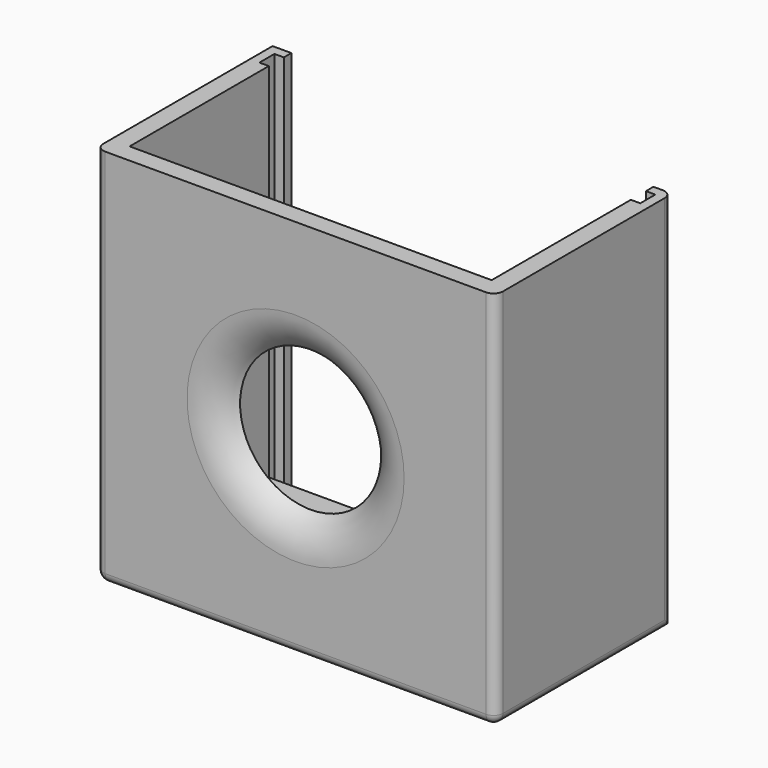
from build123d import *

# Parameters (mm, degrees)
F2_W      = 42.5
F2_H      = 40.5
F2_R      = 7.5
F8_DEPTH  = 2
F6_W      = 23.5
F6_H      = 40.5
F9_DEPTH  = 2
F5_W      = 23.5
F5_H      = 40.5
F10_DEPTH = 2
F0_W      = 42.5
F0_H      = 20.5
F11_DEPTH = 2
F7_W      = 1
F7_H      = 2
F12_DEPTH = 38.5
F13_DEPTH = 40.5
F14_R     = 0.99999


# Not quite as in the source:
# - a fillet or chamfer that OpenCascade refuses, or shapes differently, is made with other operations: its cross-section is extruded or revolved along the edge and cut away or added
# - a fillet or chamfer is up to 0.001 mm smaller than in the source, because OpenCascade refuses the exact size


with BuildPart() as f8:
    # F2 (on line) → F8 (new body)
    with BuildSketch(Plane.XZ.offset(10.25)):
        with Locations((0, 20.25)):
            Rectangle(F2_W, F2_H)
        with Locations((0, 20.25)):
            Circle(F2_R, mode=Mode.SUBTRACT)
    extrude(amount=-F8_DEPTH)

    # F6 (on line) → F9 (join)
    with BuildSketch(Plane(origin=(-21.25, 0, 0), x_dir=(0, -1, 0), z_dir=(-1, 0, 0))):
        with Locations((-1.5, 20.25)):
            Rectangle(F6_W, F6_H)
    extrude(amount=-F9_DEPTH)

    # F5 (on line) → F10 (join)
    with BuildSketch(Plane.YZ.offset(21.25)):
        with Locations((1.5, 20.25)):
            Rectangle(F5_W, F5_H)
    extrude(amount=-F10_DEPTH)

    # F0 (on Top) → F11 (join)
    with BuildSketch(Plane.XY):
        Rectangle(F0_W, F0_H)
    extrude(amount=F11_DEPTH)

    # F7 (on Top) → F12 (cut)
    with BuildSketch(Plane.XY):
        with Locations((-19.75, 11.25)):
            Rectangle(F7_W, F7_H)
        with Locations((19.75, 11.25)):
            Rectangle(F7_W, F7_H)
    extrude(amount=-F12_DEPTH, mode=Mode.SUBTRACT)

    # F7 (on Top) → F13 (cut)
    with BuildSketch(Plane.XY):
        with Locations((19.75, 11.25)):
            Rectangle(F7_W, F7_H)
        with Locations((-19.75, 11.25)):
            Rectangle(F7_W, F7_H)
    extrude(amount=F13_DEPTH, mode=Mode.SUBTRACT)

    # F14 (radius 1 in the source; OpenCascade refuses exactly that, so slightly less here)
    f14_edges = [f8.edges().sort_by_distance(p)[0] for p in [
        (0, -10.25, 0),
        (21.25, 1.5, 0),
        (21.25, 13.25, 20.25),
        (21.25, -10.25, 20.25),
        (-21.25, -10.25, 20.25),
        (-21.25, 1.5, 0),
    ]]
    fillet(f14_edges, radius=F14_R)

    # F15: fillet of radius 5.08 on 1 edges, made by hand

    # F15_s1 → F15_t2 (revolve, cut)
    with BuildSketch(Plane.XY.offset(20.25)):
        with BuildLine():
            ThreePointArc((11.5398019753, -10.25), (9.2859164414, -9.7226256161), (7.5, -8.25))
            Line((7.5, -8.25), (7.5, -10.25))
            Line((7.5, -10.25), (11.5398019753, -10.25))
        make_face()
    revolve(axis=Axis((0, -10.25, 20.25), (0, -1, 0)), mode=Mode.SUBTRACT)


solid = f8.part
